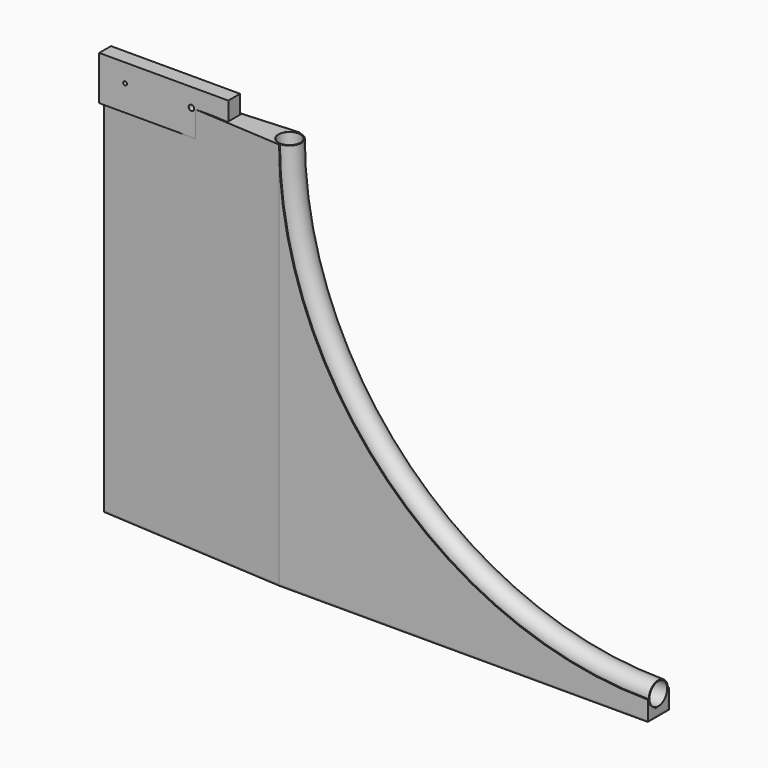
from build123d import *

# Parameters (mm, degrees)
F1_R           = 32.5
F1_R_2         = 30
F3_W           = 350
F3_H           = 120
F6_DEPTH       = 20
F5_E11_W       = 501.055137
F5_E11_H       = 1050
F9_DEPTH       = 3
F12_DEPTH      = 3
F14_DEPTH      = 3
F17_DEPTH      = 3
F0_R           = 7.5
F0_R_2         = 5
F18_DEPTH      = 35.501
F18_DEPTH_BACK = 35.501
F19_R          = 32.5
F19_R_2        = 30
F20_DEPTH      = 650


with BuildPart() as f2:
    # F2: sweep along a path in F0
    with BuildLine(Plane.XZ) as f2_path:
        ThreePointArc((250, 0), (542.893219, -707.106781), (1250, -1000))
    # F1 (on Top) → F2 (sweep)
    with BuildSketch(Plane.XY):
        with Locations((250, 0)):
            Circle(F1_R)
        with Locations((250, 0)):
            Circle(F1_R_2, mode=Mode.SUBTRACT)
    sweep(path=f2_path.line)


with BuildPart() as f6:
    # F3 (on Front) → F6 (new body, symmetric)
    with BuildSketch(Plane.XZ):
        with Locations((-75, -10)):
            Rectangle(F3_W, F3_H)
    extrude(amount=F6_DEPTH, both=True)


with BuildPart() as f9:
    # F8 (on offset) + F5_E11 (on explicit) → F9 (new body)
    with BuildSketch(Plane.XZ.offset(-32.5)):
        with BuildLine():
            Line((250, -1050), (1250, -1050))
            Line((1250, -1050), (1250, -1000))
            ThreePointArc((1250, -1000), (542.893219, -707.106781), (250, 0))
            Line((250, 0), (250, -1050))
        make_face()
    with BuildSketch(Plane(origin=(250, 32.5, 0), x_dir=(-0.997894, -0.064863, 0), z_dir=(0.064863, -0.997894, 0))):
        with Locations((250.527569, 525)):
            Rectangle(F5_E11_W, F5_E11_H)
    extrude(amount=-F9_DEPTH, dir=(0, -1, 0))


with BuildPart() as f10_1:
    # F10: instance of F9
    add(f9.part.mirror(Plane.XZ))


with BuildPart() as f12:
    # F11 (on face) → F12 (new body)
    with BuildSketch(Plane.YZ.offset(1250)):
        with BuildLine():
            Line((32.5, -1050), (32.5, -1000))
            ThreePointArc((32.5, -1000), (0, -1032.5), (-32.5, -1000))
            Line((-32.5, -1000), (-32.5, -1050))
            Line((-32.5, -1050), (32.5, -1050))
        make_face()
    extrude(amount=-F12_DEPTH)


with BuildPart() as f14:
    # F13 (on face) → F14 (new body)
    with BuildSketch(Plane(origin=(0, 0, -1050), x_dir=(1, 0, 0), z_dir=(0, 0, -1))):
        Polygon((250, -35.5), (1250, -35.5), (1250, 35.5), (250, 35.5), (-250, 3), (-250, -3), align=None)
    extrude(amount=F14_DEPTH)


with BuildPart() as f17:
    # F16 (on face) → F17 (new body)
    with BuildSketch(Plane.XY):
        with BuildLine():
            Line((245.792776, 32.22653), (250, 32.5))
            ThreePointArc((250, 32.5), (247.891949, 32.431561), (245.792776, 32.22653))
        make_face()
    extrude(amount=-F17_DEPTH)


with BuildPart() as f17b:
    # F16 (on face) → F17, piece 2 (new body)
    with BuildSketch(Plane.XY):
        with BuildLine():
            Line((250, -32.5), (245.792776, -32.22653))
            ThreePointArc((245.792776, -32.22653), (247.891949, -32.431561), (250, -32.5))
        make_face()
    extrude(amount=-F17_DEPTH)


with BuildPart() as f17c:
    # F16 (on face) → F17, piece 3 (new body)
    with BuildSketch(Plane.XY):
        with BuildLine():
            ThreePointArc((245.792776, -32.22653), (217.5, 0), (245.792776, 32.22653))
            Line((245.792776, 32.22653), (100, 22.75))
            Line((100, 22.75), (100, -22.75))
            Line((100, -22.75), (245.792776, -32.22653))
        make_face()
    extrude(amount=-F17_DEPTH)


with BuildPart() as f18_tool:
    # F0 (on Front) → F18 (new body, two sides)
    with BuildSketch(Plane.XZ) as f18_sk:
        Circle(F0_R)
        with Locations((-180, 0)):
            Circle(F0_R_2)
    extrude(amount=-F18_DEPTH)
    extrude(f18_sk.sketch, amount=F18_DEPTH_BACK)


with BuildPart() as f6_1:
    add(f6.part)

    # F18: cut by f18_tool
    add(f18_tool.part, mode=Mode.SUBTRACT)


with BuildPart() as f9_1:
    add(f9.part)

    # F18: cut by f18_tool
    add(f18_tool.part, mode=Mode.SUBTRACT)


with BuildPart() as f10_1_1:
    add(f10_1.part)

    # F18: cut by f18_tool
    add(f18_tool.part, mode=Mode.SUBTRACT)


with BuildPart() as f20:
    # F19 (on face) → F20 (new body)
    with BuildSketch(Plane.XY.offset(-1050)):
        with Locations((250, 0)):
            Circle(F19_R)
        with Locations((250, 0)):
            Circle(F19_R_2, mode=Mode.SUBTRACT)
    extrude(amount=F20_DEPTH)


solid = Compound([f2.part, f12.part, f14.part, f17.part, f17b.part, f17c.part, f6_1.part, f9_1.part, f10_1_1.part, f20.part])
